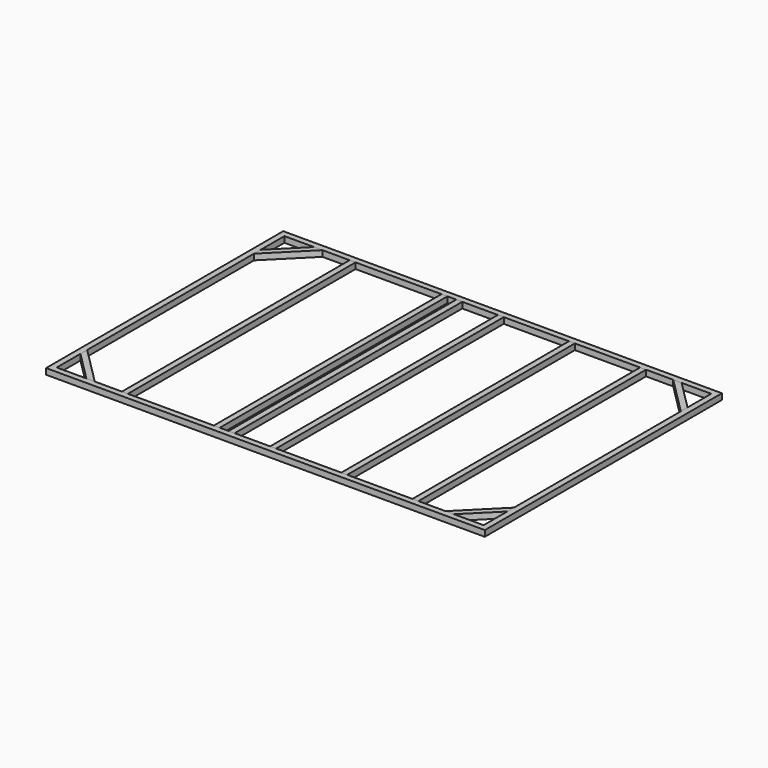
from build123d import *

# Parameters (mm, degrees)
F0_W     = 1879.6
F0_H     = 1270
F0_W_2   = 1828.8
F0_H_2   = 1219.2
F1_DEPTH = 25.4
F2_W     = 25.4
F2_H     = 1219.2
F3_DEPTH = 25.4
F5_DEPTH = 25.4
F6_T     = -3.175
F7_T     = -3.175
F8_T     = -3.175
F9_T     = -3.175
F10_T    = -3.175
F10_2_T  = -3.175
F10_3_T  = -3.175
F10_4_T  = -3.175
F10_5_T  = -3.175
F10_6_T  = -3.175


with BuildPart() as f1:
    # F0 (on Top) → F1 (new body)
    with BuildSketch(Plane.XY):
        with Locations((-914.4, 609.6)):
            Rectangle(F0_W, F0_H)
        with Locations((-914.4, 609.6)):
            Rectangle(F0_W_2, F0_H_2, mode=Mode.SUBTRACT)
    extrude(amount=F1_DEPTH)


with BuildPart() as f3:
    # F2 (on face) → F3 (new body)
    with BuildSketch(Plane.XY.offset(25.4)):
        with Locations((-1536.7, 609.6)):
            Rectangle(F2_W, F2_H)
    extrude(amount=-F3_DEPTH)

    # F10#6
    f10_6_openings = [f3.faces().sort_by_distance(p)[0] for p in [
        (-1536.7, 0, 12.7),
        (-1536.7, 1219.2, 12.7),
    ]]
    offset(amount=F10_6_T, openings=f10_6_openings)


with BuildPart() as f3b:
    # F2 (on face) → F3, piece 2 (new body)
    with BuildSketch(Plane.XY.offset(25.4)):
        with Locations((-1143, 609.6)):
            Rectangle(F2_W, F2_H)
    extrude(amount=-F3_DEPTH)

    # F10#5
    f10_5_openings = [f3b.faces().sort_by_distance(p)[0] for p in [
        (-1143, 0, 12.7),
        (-1143, 1219.2, 12.7),
    ]]
    offset(amount=F10_5_T, openings=f10_5_openings)


with BuildPart() as f3c:
    # F2 (on face) → F3, piece 3 (new body)
    with BuildSketch(Plane.XY.offset(25.4)):
        with Locations((-1079.5, 609.6)):
            Rectangle(F2_W, F2_H)
    extrude(amount=-F3_DEPTH)

    # F10#4
    f10_4_openings = [f3c.faces().sort_by_distance(p)[0] for p in [
        (-1079.5, 0, 12.7),
        (-1079.5, 1219.2, 12.7),
    ]]
    offset(amount=F10_4_T, openings=f10_4_openings)


with BuildPart() as f3d:
    # F2 (on face) → F3, piece 4 (new body)
    with BuildSketch(Plane.XY.offset(25.4)):
        with Locations((-901.7, 609.6)):
            Rectangle(F2_W, F2_H)
    extrude(amount=-F3_DEPTH)

    # F10#3
    f10_3_openings = [f3d.faces().sort_by_distance(p)[0] for p in [
        (-901.7, 1219.2, 12.7),
        (-901.7, 0, 12.7),
    ]]
    offset(amount=F10_3_T, openings=f10_3_openings)


with BuildPart() as f3e:
    # F2 (on face) → F3, piece 5 (new body)
    with BuildSketch(Plane.XY.offset(25.4)):
        with Locations((-596.9, 609.6)):
            Rectangle(F2_W, F2_H)
    extrude(amount=-F3_DEPTH)

    # F10#2
    f10_2_openings = [f3e.faces().sort_by_distance(p)[0] for p in [
        (-596.9, 0, 12.7),
        (-596.9, 1219.2, 12.7),
    ]]
    offset(amount=F10_2_T, openings=f10_2_openings)


with BuildPart() as f3f:
    # F2 (on face) → F3, piece 6 (new body)
    with BuildSketch(Plane.XY.offset(25.4)):
        with Locations((-292.1, 609.6)):
            Rectangle(F2_W, F2_H)
    extrude(amount=-F3_DEPTH)

    # F10
    f10_openings = [f3f.faces().sort_by_distance(p)[0] for p in [
        (-292.1, 1219.2, 12.7),
        (-292.1, 0, 12.7),
    ]]
    offset(amount=F10_T, openings=f10_openings)


with BuildPart() as f5:
    # F4 (on face) → F5 (new body)
    with BuildSketch(Plane(origin=(0, 0, 0), x_dir=(1, 0, 0), z_dir=(0, 0, -1))):
        Polygon((-1665.8789755157, 0), (-1701.8, 0), (-1828.8, -127), (-1828.8, -162.9210244843), align=None)
    extrude(amount=-F5_DEPTH)

    # F7
    f7_openings = [f5.faces().sort_by_distance(p)[0] for p in [
        (-1828.8, 144.960512, 12.7),
        (-1683.839488, 0, 12.7),
    ]]
    offset(amount=F7_T, openings=f7_openings, kind=Kind.INTERSECTION)


with BuildPart() as f5b:
    # F4 (on face) → F5, piece 2 (new body)
    with BuildSketch(Plane(origin=(0, 0, 0), x_dir=(1, 0, 0), z_dir=(0, 0, -1))):
        Polygon((-1665.8789755157, -1219.2), (-1828.8, -1056.2789755157), (-1828.8, -1092.2), (-1701.8, -1219.2), align=None)
    extrude(amount=-F5_DEPTH)

    # F6
    f6_openings = [f5b.faces().sort_by_distance(p)[0] for p in [
        (-1828.8, 1074.239488, 12.7),
        (-1683.839488, 1219.2, 12.7),
    ]]
    offset(amount=F6_T, openings=f6_openings, kind=Kind.INTERSECTION)


with BuildPart() as f5c:
    # F4 (on face) → F5, piece 3 (new body)
    with BuildSketch(Plane(origin=(0, 0, 0), x_dir=(1, 0, 0), z_dir=(0, 0, -1))):
        Polygon((0, -1092.2), (0, -1056.2789755157), (-162.9210244843, -1219.2), (-127, -1219.2), align=None)
    extrude(amount=-F5_DEPTH)

    # F9
    f9_openings = [f5c.faces().sort_by_distance(p)[0] for p in [
        (0, 1074.239488, 12.7),
        (-144.960512, 1219.2, 12.7),
    ]]
    offset(amount=F9_T, openings=f9_openings, kind=Kind.INTERSECTION)


with BuildPart() as f5d:
    # F4 (on face) → F5, piece 4 (new body)
    with BuildSketch(Plane(origin=(0, 0, 0), x_dir=(1, 0, 0), z_dir=(0, 0, -1))):
        Polygon((-127, 0), (-162.9210244843, 0), (0, -162.9210244843), (0, -127), align=None)
    extrude(amount=-F5_DEPTH)

    # F8
    f8_openings = [f5d.faces().sort_by_distance(p)[0] for p in [
        (0, 144.960512, 12.7),
        (-144.960512, 0, 12.7),
    ]]
    offset(amount=F8_T, openings=f8_openings, kind=Kind.INTERSECTION)


solid = Compound([f1.part, f3.part, f3b.part, f3c.part, f3d.part, f3e.part, f3f.part, f5.part, f5b.part, f5c.part, f5d.part])
